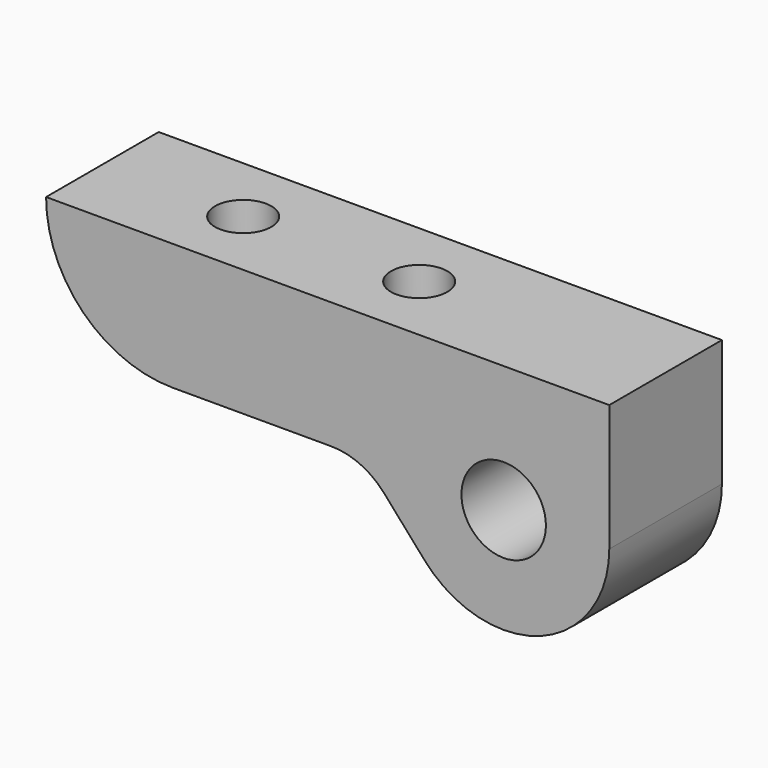
from build123d import *

# Parameters (mm, degrees)
F0_R     = 6
F1_DEPTH = 20
F2_R     = 10
F4_D     = 8
F4_DEPTH = 10
F4_TIP   = 2.4034424761
F5_R     = 17.99999


# Not quite as in the source:
# - a fillet or chamfer is up to 0.001 mm smaller than in the source, because OpenCascade refuses the exact size


with BuildPart() as f1:
    # F0 (on Front) → F1 (new body)
    with BuildSketch(Plane.XZ):
        with BuildLine():
            Line((-20, 0), (-11.25, -9.9215674165))
            ThreePointArc((-11.25, -9.9215674165), (5.3033008589, -14.0312152004), (15, 0))
            Line((15, 0), (15, 15))
            Line((15, 15), (15, 18))
            Line((15, 18), (-65, 18))
            Line((-65, 18), (-65, 0))
            Line((-65, 0), (-20, 0))
        make_face()
        Circle(F0_R, mode=Mode.SUBTRACT)
    extrude(amount=F1_DEPTH)

    # F2
    f2_edges = [f1.edges().sort_by_distance(p)[0] for p in [
        (-20, -10, 0),
    ]]
    fillet(f2_edges, radius=F2_R)

    # F4
    with Locations(Plane.XY.offset(18)):
        with Locations((-45, -10), (-20, -10)):
            Hole(F4_D / 2, depth=F4_DEPTH)
            with Locations((0, 0, -(F4_DEPTH + F4_TIP / 2))):  # 118° drill point
                Cone(0, F4_D / 2, F4_TIP, mode=Mode.SUBTRACT)

    # F5 (radius 18 in the source; OpenCascade refuses exactly that, so slightly less here)
    f5_edges = [f1.edges().sort_by_distance(p)[0] for p in [
        (-65, -10, 0),
    ]]
    fillet(f5_edges, radius=F5_R)


solid = f1.part
